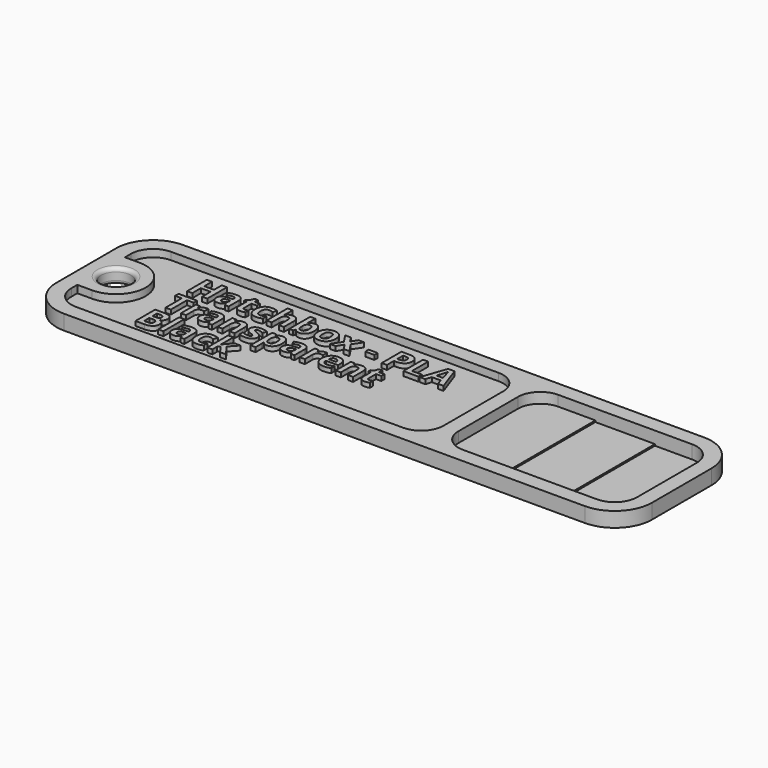
from build123d import *

# Parameters (mm, degrees)
F1_DEPTH      = 2
F3_DEPTH      = 1
F4_R          = 2
F5_DEPTH      = 2.001
F6_R          = 0.5
F7_DEPTH      = 0.4
F9_DEPTH      = 0.2
F11_DEPTH     = 0.2
F12_TEXT_SIZE = 4.6296296296
F13_DEPTH     = 0.6


# Not quite as in the source:
# - Text() gives the source's letters only with a copy of the font that has no kerning and outlines rounded to 1/6400 em; it was checked with that copy


with BuildPart() as f1:
    # F0 (on Top) → F1 (new body)
    with BuildSketch(Plane.XY):
        with BuildLine():
            ThreePointArc((40, 5), (38.5355339059, 8.5355339059), (35, 10))
            Line((35, 10), (-35, 10))
            ThreePointArc((-35, 10), (-38.5355339059, 8.5355339059), (-40, 5))
            Line((-40, 5), (-40, -5))
            ThreePointArc((-40, -5), (-38.5355339059, -8.5355339059), (-35, -10))
            Line((-35, -10), (35, -10))
            ThreePointArc((35, -10), (38.5355339059, -8.5355339059), (40, -5))
            Line((40, -5), (40, 5))
        make_face()
    extrude(amount=F1_DEPTH)

    # F2 (on face) → F3 (cut)
    with BuildSketch(Plane.XY.offset(2)):
        with BuildLine():
            ThreePointArc((35, -8), (37.1213203436, -7.1213203436), (38, -5))
            Line((38, -5), (38, 5))
            ThreePointArc((38, 5), (37.1213203436, 7.1213203436), (35, 8))
            Line((35, 8), (17, 8))
            ThreePointArc((17, 8), (14.8786796564, 7.1213203436), (14, 5))
            Line((14, 5), (14, -5))
            ThreePointArc((14, -5), (14.8786796564, -7.1213203436), (17, -8))
            Line((17, -8), (35, -8))
        make_face()
        with BuildLine():
            ThreePointArc((-38, -5), (-37.1213203436, -7.1213203436), (-35, -8))
            Line((-35, -8), (9, -8))
            ThreePointArc((9, -8), (11.1213203436, -7.1213203436), (12, -5))
            Line((12, -5), (12, 5))
            ThreePointArc((12, 5), (11.1213203436, 7.1213203436), (9, 8))
            Line((9, 8), (-35, 8))
            ThreePointArc((-35, 8), (-37.1213203436, 7.1213203436), (-38, 5))
            Line((-38, 5), (-38, 4))
            Line((-38, 4), (-36, 4))
            ThreePointArc((-36, 4), (-32, 0), (-36, -4))
            Line((-36, -4), (-38, -4))
            Line((-38, -4), (-38, -5))
        make_face()
    extrude(amount=-F3_DEPTH, mode=Mode.SUBTRACT)

    # F4 (on face) → F5 (cut, through all)
    with BuildSketch(Plane.XY.offset(2)):
        with Locations((-36, 0)):
            Circle(F4_R)
    extrude(amount=-F5_DEPTH, mode=Mode.SUBTRACT)

    # F6
    f6_edges = [f1.edges().sort_by_distance(p)[0] for p in [
        (-38, 0, 2),
        (-38, 0, 0),
    ]]
    fillet(f6_edges, radius=F6_R)

    # F7 (cut): a face of the model
    f7_faces = [f1.faces().sort_by_distance(p)[0] for p in [
        (26, 0, 1),
    ]]
    extrude(f7_faces, amount=-F7_DEPTH, mode=Mode.SUBTRACT)

    # F8 (on face) → F9 (cut)
    with BuildSketch(Plane.XY.offset(0.6)):
        with BuildLine():
            Line((22, -8), (35, -8))
            ThreePointArc((35, -8), (37.1213203436, -7.1213203436), (38, -5))
            Line((38, -5), (38, 5))
            ThreePointArc((38, 5), (37.1213203436, 7.1213203436), (35, 8))
            Line((35, 8), (22, 8))
            Line((22, 8), (22, -8))
        make_face()
    extrude(amount=-F9_DEPTH, mode=Mode.SUBTRACT)

    # F10 (on face) → F11 (cut)
    with BuildSketch(Plane.XY.offset(0.4)):
        with BuildLine():
            ThreePointArc((38, 5), (37.1213203436, 7.1213203436), (35, 8))
            Line((35, 8), (30, 8))
            Line((30, 8), (30, -8))
            Line((30, -8), (35, -8))
            ThreePointArc((35, -8), (37.1213203436, -7.1213203436), (38, -5))
            Line((38, -5), (38, 5))
        make_face()
    extrude(amount=-F11_DEPTH, mode=Mode.SUBTRACT)

    # F12 (on face) → F13 (join)
    with BuildSketch(Plane.XY.offset(1)):
        with Locations((-29, 2.6666666667)):
            Text('Hatchbox - PLA', F12_TEXT_SIZE, font='Open Sans', font_style=FontStyle.BOLD, text_align=(TextAlign.LEFT, TextAlign.BOTTOM))
        with Locations((-29, -1.6666666667)):
            Text('Transparent', F12_TEXT_SIZE, font='Open Sans', font_style=FontStyle.BOLD, text_align=(TextAlign.LEFT, TextAlign.BOTTOM))
        with Locations((-29, -6)):
            Text('Black', F12_TEXT_SIZE, font='Open Sans', font_style=FontStyle.BOLD, text_align=(TextAlign.LEFT, TextAlign.BOTTOM))
    extrude(amount=F13_DEPTH)


solid = f1.part
